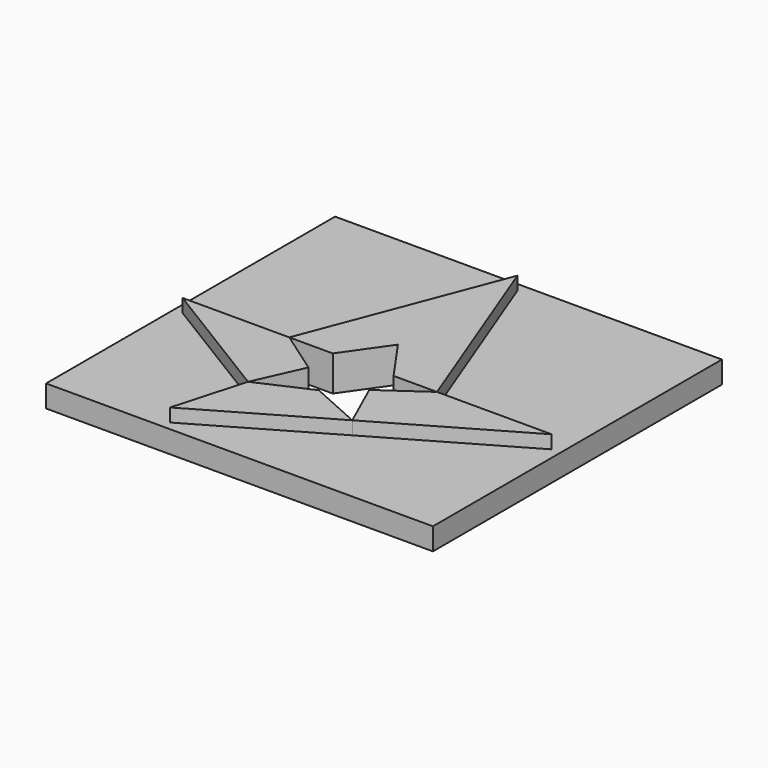
from build123d import *

# Parameters (mm, degrees)
F1_DEPTH = 6.35
F2_DEPTH = 10.16


# Not quite as in the source:
# - a feature names something its author has since deleted; it is built from what else it names


with BuildPart() as f1:
    # F0 (on Top) → F1 (new body)
    with BuildSketch(Plane.XY):
        Polygon((56.7444791493, 57.9814615035), (-51.9109388844, 57.9814615035), (-54.4509388844, 57.9814615035), (-54.4509388844, -45.8724710478), (-51.9109388844, -45.8724710478), (56.7444791493, -45.8724710478), align=None)
        Polygon((-51.9109388844, 0), (-21.225182045, 0), (0, 55.4414615035), (21.225182045, 0), (54.2044791493, 0), (14.9832434675, -22.6443909789), (-20.8495623229, -43.3324710478), (-14.9832434675, -22.6443909789), align=None, mode=Mode.SUBTRACT)
    extrude(amount=F1_DEPTH)


with BuildPart() as f2:
    # F0 (on Top) → F2 (new body)
    with BuildSketch(Plane.XY):
        Polygon((-8.74130489, 0), (0, 12.483877155), (8.74130489, 0), (21.225182045, 0), (0, 55.4414615035), (-21.225182045, 0), align=None)
    extrude(amount=F2_DEPTH)


with BuildPart() as f2b:
    # F0 (on Top) → F2, piece 2 (new body)
    with BuildSketch(Plane.XY):
        Polygon((-8.74130489, -8.74130489), (-21.225182045, 0), (-51.9109388844, 0), (-14.9832434675, -22.6443909789), align=None)
    extrude(amount=F2_DEPTH)


with BuildPart() as f2c:
    # F0 (on Top) → F2, piece 3 (new body)
    with BuildSketch(Plane.XY):
        Polygon((0, -15.9175042418), (-14.9832434675, -22.6443909789), (-20.8495623229, -43.3324710478), (14.9832434675, -22.6443909789), align=None)
    extrude(amount=F2_DEPTH)


with BuildPart() as f2d:
    # F0 (on Top) → F2, piece 4 (new body)
    with BuildSketch(Plane.XY):
        Polygon((54.2044791493, 0), (21.225182045, 0), (8.74130489, -8.74130489), (14.9832434675, -22.6443909789), align=None)
    extrude(amount=F2_DEPTH)


solid = Compound([f1.part, f2.part, f2b.part, f2c.part, f2d.part])
